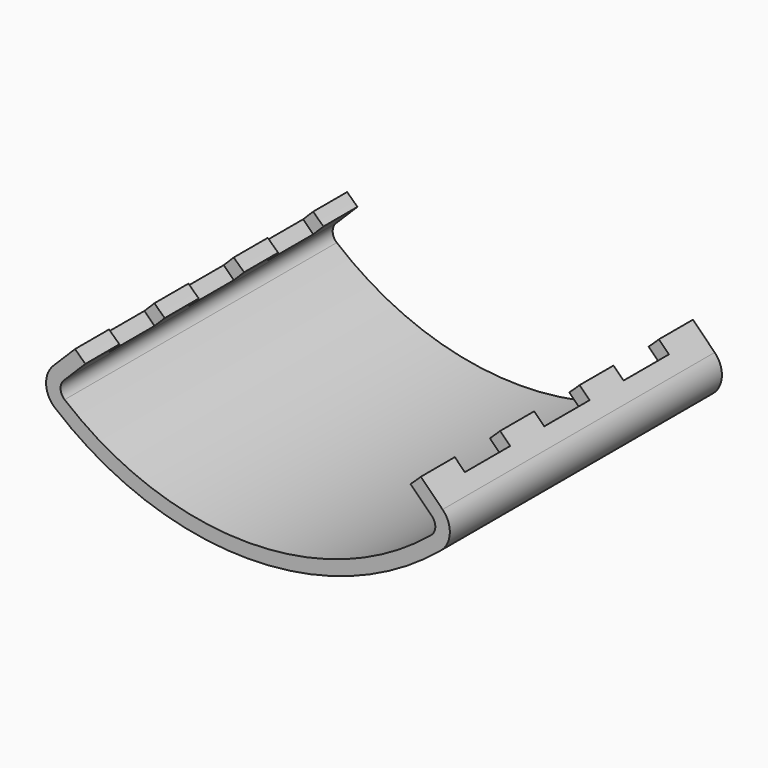
from build123d import *

# Parameters (mm, degrees)
F1_DEPTH = 76.2
F2_R     = 11.1125
F3_R     = 5.08
F4_W     = 25.4
F4_H     = 9.6059094062
F4_H_2   = 10.5453204632
F5_DEPTH = 25.4
F6_W     = 25.4
F6_H     = 12.6698460698
F6_H_2   = 15.3897032142
F7_DEPTH = 25.4


with BuildPart() as f1:
    # F0 (on Front) → F1 (new body, symmetric)
    with BuildSketch(Plane.XZ):
        with BuildLine():
            ThreePointArc((85.5011615648, -96.0432013591), (0, -128.5875), (-85.5011615648, -96.0432013591))
            ThreePointArc((-85.5011615648, -96.0432013591), (-85.91339025, -95.6746284654), (-86.3240301315, -95.3042862526))
            Line((-86.3240301315, -95.3042862526), (-72.8343228145, -81.8145789356))
            ThreePointArc((-72.8343228145, -81.8145789356), (-75.1761291277, -79.6681461792), (-77.4547090442, -77.4547090442))
            Line((-77.4547090442, -77.4547090442), (-90.9250932258, -90.9250932258))
            Line((-90.9250932258, -90.9250932258), (-95.4152212864, -95.4152212864))
            ThreePointArc((-95.4152212864, -95.4152212864), (0, -134.9375), (95.4152212864, -95.4152212864))
            Line((95.4152212864, -95.4152212864), (77.4547090442, -77.4547090442))
            ThreePointArc((77.4547090442, -77.4547090442), (75.1761291277, -79.6681461792), (72.8343228145, -81.8145789356))
            Line((72.8343228145, -81.8145789356), (86.3240301315, -95.3042862526))
            ThreePointArc((86.3240301315, -95.3042862526), (85.91339025, -95.6746284654), (85.5011615648, -96.0432013591))
        make_face()
    extrude(amount=F1_DEPTH, both=True)

    # F2
    f2_edges = [f1.edges().sort_by_distance(p)[0] for p in [
        (95.415221, 0, -95.415221),
        (-95.415221, 0, -95.415221),
    ]]
    fillet(f2_edges, radius=F2_R)

    # F3
    f3_edges = [f1.edges().sort_by_distance(p)[0] for p in [
        (-86.32403, 0, -95.304286),
        (86.32403, 0, -95.304286),
    ]]
    fillet(f3_edges, radius=F3_R)

    # F4 (on face) → F5 (cut)
    with BuildSketch(Plane(origin=(0, 0, 0), x_dir=(0, 1, 0), z_dir=(0.7071067812, 0, 0.7071067812))):
        with Locations((-44.45, -111.0845452969)):
            Rectangle(F4_W, F4_H)
        with Locations((44.45, -111.0845452969)):
            Rectangle(F4_W, F4_H)
        with Locations((0, -110.6148397684)):
            Rectangle(F4_W, F4_H_2)
    extrude(amount=-F5_DEPTH, mode=Mode.SUBTRACT)

    # F6 (on face) → F7 (cut)
    with BuildSketch(Plane(origin=(0, 0, 0), x_dir=(0, -1, 0), z_dir=(-0.7071067812, 0, 0.7071067812))):
        with Locations((-44.45, -109.5525769651)):
            Rectangle(F6_W, F6_H)
        with Locations((44.45, -109.5525769651)):
            Rectangle(F6_W, F6_H)
        with Locations((0, -108.1926483929)):
            Rectangle(F6_W, F6_H_2)
    extrude(amount=-F7_DEPTH, mode=Mode.SUBTRACT)


solid = f1.part
